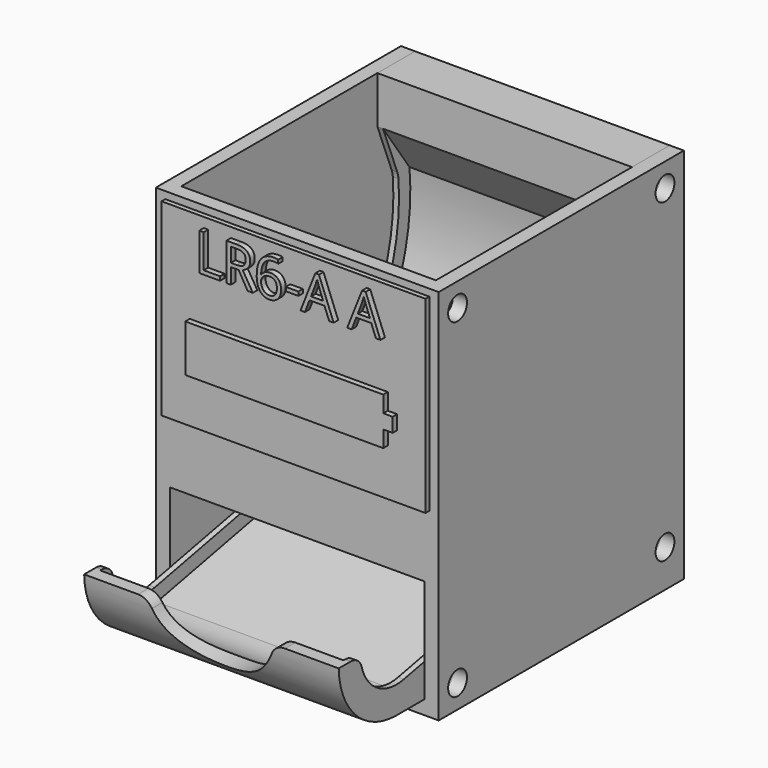
from build123d import *

# Parameters (mm, degrees)
F1_DEPTH     = 80
F2_W         = 54
F2_H         = 22
F3_DEPTH     = 65.001
F4_DEPTH     = 11.8
F5_W         = 56
F5_H         = 40
F6_DEPTH     = 1
F7_DEPTH     = 1
F10_DEPTH    = 1.2
F8_TEXT_SIZE = 11.1111111111
F11_DEPTH    = 1.2
F12_W        = 54
F12_H        = 3
F13_DEPTH    = 15
F15_DEPTH    = 27
F16_R        = 2.5
F17_DEPTH    = 30
F18_W        = 1.2
F18_H        = 3
F22_DEPTH    = 22.7580585408
F23_R        = 3.1
F24_R        = 3
F26_DEPTH    = 1.2
F28_DEPTH    = 1.2
F29_R        = 5


# Not quite as in the source:
# - Text() gives the source's letters only with a copy of the font that has no kerning and outlines rounded to 1/6400 em; it was checked with that copy


with BuildPart() as f1:
    # F0 (on Top) → F1 (new body)
    with BuildSketch(Plane.XY):
        Polygon((-27, 65), (-30, 65), (-30, 0), (30, 0), (30, 65), (27, 65), (27, 3), (-27, 3), align=None)
    extrude(amount=F1_DEPTH)

    # F2 (on face) → F3 (cut, through all)
    with BuildSketch(Plane.XZ):
        with Locations((0, 14)):
            Rectangle(F2_W, F2_H)
    extrude(amount=-F3_DEPTH, mode=Mode.SUBTRACT)

    # F4 (add): a face of the model
    f4_faces = [f1.faces().sort_by_distance(p)[0] for p in [
        (0, 3, 1.5),
    ]]
    extrude(f4_faces, amount=F4_DEPTH)

    # F5 (on face) → F6 (cut)
    with BuildSketch(Plane.XZ):
        with Locations((0, 58.5)):
            Rectangle(F5_W, F5_H)
    extrude(amount=-F6_DEPTH, mode=Mode.SUBTRACT)

    # F12 (on face) → F13 (join)
    with BuildSketch(Plane(origin=(0, 65, 0), x_dir=(-1, 0, 0), z_dir=(0, 1, 0))):
        with Locations((0, 1.5)):
            Rectangle(F12_W, F12_H)
    extrude(amount=-F13_DEPTH)


with BuildPart() as f7:
    # F5 (on face) → F7 (new body)
    with BuildSketch(Plane.XZ):
        with Locations((0, 58.5)):
            Rectangle(F5_W, F5_H)
    extrude(amount=F7_DEPTH)

    # F9 (on face) → F10 (join)
    with BuildSketch(Plane.XZ.offset(1)):
        Polygon((20, 58.5), (-22, 58.5), (-22, 48.5), (20, 48.5), (20, 52), (22, 52), (22, 55), (20, 55), align=None)
    extrude(amount=F10_DEPTH)

    # F8 (on face) → F11 (join)
    with BuildSketch(Plane.XZ.offset(1)):
        with Locations((-20.1163194444, 68.5)):
            Text('LR6-A A', F8_TEXT_SIZE, font='Open Sans', text_align=(TextAlign.LEFT, TextAlign.BOTTOM))
    extrude(amount=F11_DEPTH)


with BuildPart() as f15:
    # F14 (on Right) → F15 (new body, symmetric)
    with BuildSketch(Plane.YZ):
        with BuildLine():
            Line((65, 3), (65, 80))
            Line((65, 80), (55, 80))
            Line((55, 80), (55, 70))
            Line((55, 70), (62, 60))
            ThreePointArc((62, 60), (53.6346037836, 29.3936067514), (26.8580673021, 12.3716134604))
            Line((26.8580673021, 12.3716134604), (-5, 6))
            ThreePointArc((-5, 6), (-15.2959173043, 8.5051033696), (-20, 18))
            Line((-20, 18), (-22.7570585408, 18))
            ThreePointArc((-22.7570585408, 18), (-18.1721426428, 7.3757151264), (-7.46, 3))
            Line((-7.46, 3), (65, 3))
        make_face()
    extrude(amount=F15_DEPTH, both=True)


with BuildPart() as f17_tool:
    # F16 (on Right) → F17 (new body, symmetric)
    with BuildSketch(Plane.YZ):
        with Locations((60, 75)):
            Circle(F16_R)
        with Locations((60, 8)):
            Circle(F16_R)
        with Locations((5, 75)):
            Circle(F16_R)
        with Locations((5, 5)):
            Circle(F16_R)
    extrude(amount=F17_DEPTH, both=True)


with BuildPart() as f1_1:
    add(f1.part)

    # F17: cut by f17_tool
    add(f17_tool.part, mode=Mode.SUBTRACT)


with BuildPart() as f15_1:
    add(f15.part)

    # F17: cut by f17_tool
    add(f17_tool.part, mode=Mode.SUBTRACT)

    # F19: sweep along a path in F19_path
    with BuildLine(Plane(origin=(27, -5, 6), x_dir=(0, 0, -1), z_dir=(-1, 0, 0))) as f19_path:
        ThreePointArc((-12, 15), (-2.5051033696, 10.2959173043), (0, 0))
        Line((0, 0), (-6.3716134604, -31.8580673021))
        ThreePointArc((-6.3716134604, -31.8580673021), (-23.3936067514, -58.6346037836), (-54, -67))
    # F18 (on face) → F19 (sweep)
    with BuildSketch(Plane.XY.offset(18)):
        with Locations((26.4, -18.5)):
            Rectangle(F18_W, F18_H)
    sweep(path=f19_path.line)

    # F20: sweep along a path in F20_path
    with BuildLine(Plane(origin=(-27, -5, 6), x_dir=(0, 0, -1), z_dir=(-1, 0, 0))) as f20_path:
        ThreePointArc((-12, 15), (-2.5051033696, 10.2959173043), (0, 0))
        Line((0, 0), (-6.3716134604, -31.8580673021))
        ThreePointArc((-6.3716134604, -31.8580673021), (-23.3936067514, -58.6346037836), (-54, -67))
    # F18 (on face) → F20 (sweep)
    with BuildSketch(Plane.XY.offset(18)):
        with Locations((-26.4, -18.5)):
            Rectangle(F18_W, F18_H)
    sweep(path=f20_path.line)

    # F21 (on Front) → F22 (cut, through all)
    with BuildSketch(Plane.XZ):
        with BuildLine():
            Line((13.416407865, 18), (-13.416407865, 18))
            ThreePointArc((-13.416407865, 18), (0, 8), (13.416407865, 18))
        make_face()
    extrude(amount=F22_DEPTH, mode=Mode.SUBTRACT)

    # F23
    f23_edges = [f15_1.edges().sort_by_distance(p)[0] for p in [
        (13.416408, -21.378529, 18),
        (-13.416408, -21.378529, 18),
    ]]
    fillet(f23_edges, radius=F23_R)

    # F24
    f24_edges = [f15_1.edges().sort_by_distance(p)[0] for p in [
        (-26.4, -17, 18),
        (26.4, -17, 18),
    ]]
    fillet(f24_edges, radius=F24_R)

    # F25 (on face) → F26 (join)
    with BuildSketch(Plane.YZ.offset(27)):
        Polygon((55, 70), (59.0091543313, 59.7658159141), (62, 60), align=None)
    extrude(amount=-F26_DEPTH)

    # F27 (on face) → F28 (join)
    with BuildSketch(Plane(origin=(-27, 0, 0), x_dir=(0, -1, 0), z_dir=(-1, 0, 0))):
        Polygon((-59.0091543313, 59.7658159141), (-55, 70), (-62, 60), align=None)
    extrude(amount=-F28_DEPTH)

    # F29
    f29_edges = [f15_1.edges().sort_by_distance(p)[0] for p in [
        (26.4, 59.009154, 59.765816),
        (-26.4, 59.009154, 59.765816),
    ]]
    fillet(f29_edges, radius=F29_R)


solid = Compound([f7.part, f1_1.part, f15_1.part])
